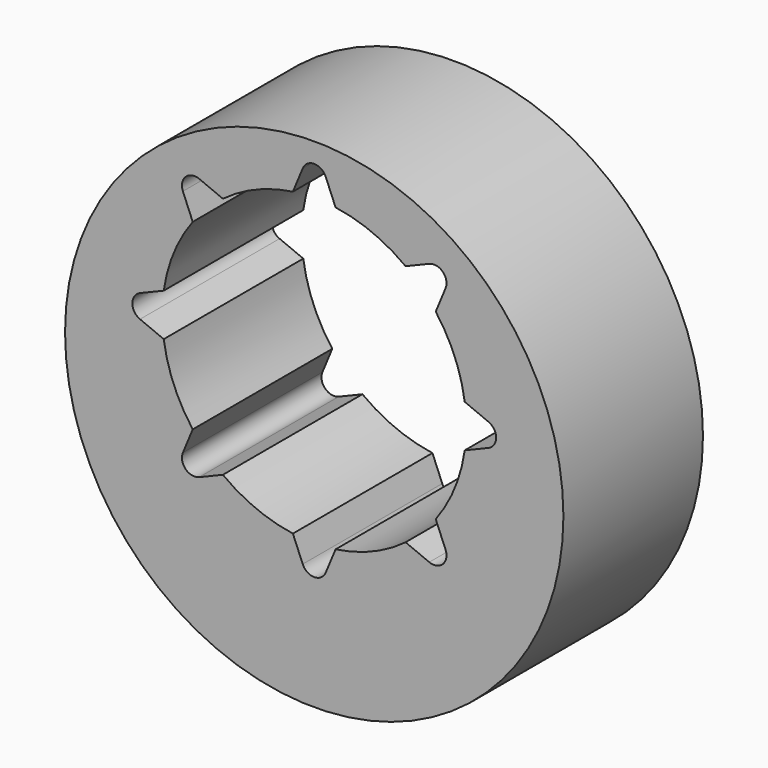
from build123d import *

# Parameters (mm, degrees)
F0_R            = 10
F0_R_2          = 6.1
F1_DEPTH        = 7
F3_DEPTH        = 7
F3_COPIES_COUNT = 8
F4_W            = 0.8
F4_H            = 2
F5_DEPTH        = 0.6
F6_T1_DEPTH     = 3.25


# Not quite as in the source:
# - a fillet or chamfer that OpenCascade refuses, or shapes differently, is made with other operations: its cross-section is extruded or revolved along the edge and cut away or added
# - a pattern or mirror of a feature is missing from the dataset's text; its kind, count and spacing are read off the source's solid


with BuildPart() as f1:
    # F0 (on Front) → F1 (new body)
    with BuildSketch(Plane.XZ):
        with Locations((0, -1.9)):
            Circle(F0_R)
        Circle(F0_R_2, mode=Mode.SUBTRACT)
    extrude(amount=F1_DEPTH)

    # F2 (on face) → F3 (cut)
    with BuildSketch(Plane.XZ.offset(7)):
        with BuildLine():
            Line((6.9913417162, 0.4619397663), (6.0396188995, 0.8561562646))
            ThreePointArc((6.0396188995, 0.8561562646), (6.0848860008, 0.429141418), (6.1, 0))
            ThreePointArc((6.1, 0), (6.0848860008, -0.429141418), (6.0396188995, -0.8561562646))
            Line((6.0396188995, -0.8561562646), (6.9913417162, -0.4619397663))
            ThreePointArc((6.9913417162, -0.4619397663), (7.3, 0), (6.9913417162, 0.4619397663))
        make_face()
    f3 = extrude(amount=-F3_DEPTH, mode=Mode.SUBTRACT)

    # F3_copies: F3 ×8 about axis
    f3_copies_axis = Axis((0, 0, 0), (0, 1, 0))
    for i in range(1, F3_COPIES_COUNT):
        add(f3.rotate(f3_copies_axis, i * 360 / F3_COPIES_COUNT), mode=Mode.SUBTRACT)

    # F4 (on face) → F5 (cut)
    with BuildSketch(Plane(origin=(0, 0, 0), x_dir=(-1, 0, 0), z_dir=(0, 1, 0))):
        with Locations((0, -9.3)):
            Rectangle(F4_W, F4_H)
    extrude(amount=-F5_DEPTH, mode=Mode.SUBTRACT)

    # F6: fillet of radius 0.5 on 2 edges, made by hand

    # F6_s2 → F6_t1 (join)
    with BuildSketch(Plane.XY.offset(-11.55)):
        with BuildLine():
            ThreePointArc((0.4, -0.1), (0.2535533906, -0.4535533906), (-0.1, -0.6))
            Line((-0.1, -0.6), (0.4, -0.6))
            Line((0.4, -0.6), (0.4, -0.1))
        make_face()
        with BuildLine():
            ThreePointArc((-0.4, -0.1), (-0.2535533906, -0.4535533906), (0.1, -0.6))
            Line((0.1, -0.6), (-0.4, -0.6))
            Line((-0.4, -0.6), (-0.4, -0.1))
        make_face()
    extrude(amount=F6_T1_DEPTH)


solid = f1.part
